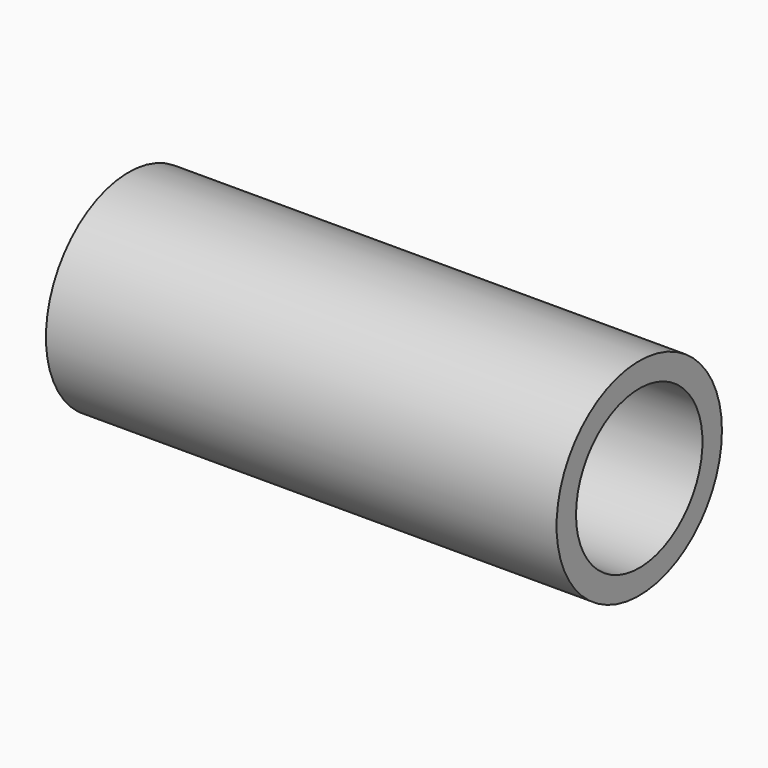
from build123d import *

# Parameters (mm, degrees)
F0_R     = 4.25
F1_DEPTH = 21
F2_R     = 4.25
F3_DEPTH = 21
F5_D     = 8.4
F4_R     = 4.2
F7_DEPTH = 21
F8_D     = 6.5


# Not quite as in the source:
# - a feature names something its author has since deleted; it is built from what else it names


with BuildPart() as f1:
    # F0 (on Right) → F1 (new body)
    with BuildSketch(Plane.YZ):
        Circle(F0_R)
    extrude(amount=F1_DEPTH)

    # F2 (on Right) → F3 (join)
    with BuildSketch(Plane.YZ):
        Circle(F2_R)
    extrude(amount=F3_DEPTH)

    # F5 (through all)
    with Locations(Plane(origin=(0, 0, 0), x_dir=(0, 1, 0), z_dir=(-1, 0, 0))):
        with Locations((0, 0)):
            Hole(F5_D / 2)

    # F4 (on face) → F7 (join)
    with BuildSketch(Plane.YZ):
        Circle(F4_R)
    extrude(amount=F7_DEPTH)

    # F8 (through all)
    with Locations(Plane(origin=(0, 0, 0), x_dir=(0, 1, 0), z_dir=(-1, 0, 0))):
        with Locations((0, 0)):
            Hole(F8_D / 2)


solid = f1.part
